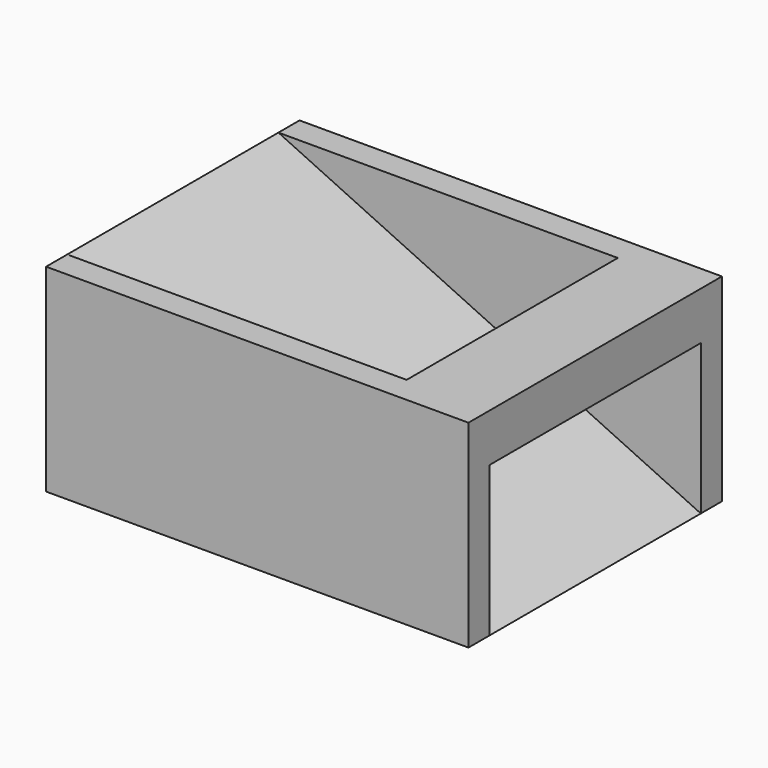
from build123d import *

# Parameters (mm, degrees)
F1_DEPTH = 38.1
F2_W     = 101.6
F2_H     = 47.625
F3_DEPTH = 6.35
F4_W     = 101.6
F4_H     = 47.625
F5_DEPTH = 6.35


# Not quite as in the source:
# - a feature names something its author has since deleted; it is built from what else it names


with BuildPart() as f1:
    # F0 (on Front) → F1 (new body, symmetric)
    with BuildSketch(Plane.XZ):
        Polygon((50.8, 12.2875440849), (50.8, 23.8125), (30.8381908, 23.8125), align=None)
    extrude(amount=F1_DEPTH, both=True)



with BuildPart() as f1b:
    # F0 (on Front) → F1, piece 2 (new body, symmetric)
    with BuildSketch(Plane.XZ):
        Polygon((50.8, -23.8125), (-50.8, 23.8125), (-50.8, -23.8125), align=None)
    extrude(amount=F1_DEPTH, both=True)


with BuildPart() as f1_1:
    add(f1.part)

    add(f1b.part)  # F3 merges F1b
    # F2 (on face) → F3 (join)
    with BuildSketch(Plane(origin=(0, 38.1, 0), x_dir=(-1, 0, 0), z_dir=(0, 1, 0))):
        Rectangle(F2_W, F2_H)
    extrude(amount=-F3_DEPTH)

    # F4 (on face) → F5 (join)
    with BuildSketch(Plane.XZ.offset(38.1)):
        Rectangle(F4_W, F4_H)
    extrude(amount=-F5_DEPTH)


solid = f1_1.part
